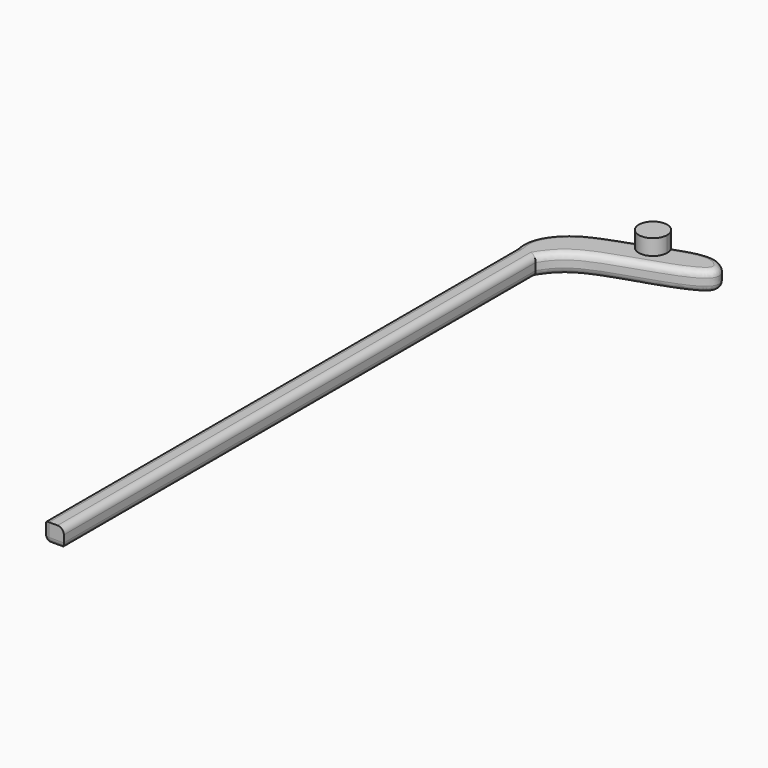
from build123d import *

# Parameters (mm, degrees)
F0_W     = 6.8017598242
F0_H     = 190.8443272114
F1_DEPTH = 6.35
F2_R     = 2.032
F4_DEPTH = 5.08


with BuildPart() as f1:
    # F0 (on Top) → F1 (new body)
    with BuildSketch(Plane.XY):
        with BuildLine():
            add(Edge.make_bspline(
                [(-18.7212117016, 95.2281802893), (-19.0287577276, 97.276144289), (-19.7432919814, 102.0342608203), (-12.2874624611, 112.4930440931), (5.2710494303, 117.2298121441), (24.2765167775, 126.2039152993), (34.1874650886, 113.5896617546), (-5.0813319368, 105.699253631), (-10.0400502329, 98.10603191), (-11.9194518775, 95.2281802893)],
                knots=[0, 0, 0, 0, 0.0947219775, 0.2200713026, 0.3846456115, 0.5513063344, 0.6487683321, 0.8668823782, 1, 1, 1, 1], degree=3))
            Line((-18.7212117016, 95.2281802893), (-11.9194518775, 95.2281802893))
        make_face()
        with Locations((-15.3203317896, -0.1939833164)):
            Rectangle(F0_W, F0_H)
    extrude(amount=F1_DEPTH)

    # F2
    f2_edges = [f1.edges().sort_by_distance(p)[0] for p in [
        (-11.919452, -0.193983, 0),
        (23.633961, 122.958027, 0),
        (-15.320332, -95.616147, 0),
        (-18.721212, -0.193983, 0),
        (-18.721212, 95.22818, 3.175),
        (-18.721212, -95.616147, 3.175),
        (-18.721212, -0.193983, 6.35),
        (-11.919452, -0.193983, 6.35),
        (19.705715, 122.814147, 6.35),
    ]]
    fillet(f2_edges, radius=F2_R)

    # F3 (on face) → F4 (join)
    with BuildSketch(Plane.XY.offset(6.35)):
        with BuildLine():
            add(Edge.make_bspline(
                [(4.3073198253, 115.4028172782), (4.4655770028, 115.4600073559), (4.6241664565, 115.5174753315), (4.7830828302, 115.5752301503), (4.9423207723, 115.633280776), (5.1018749356, 115.6916361901), (5.2617399779, 115.7503053906), (5.4219105623, 115.809297391), (5.5823813583, 115.8686212189), (5.7431470418, 115.9282859145), (5.9042022968, 115.9883005294), (6.065541816, 116.0486741248), (6.2271603024, 116.1094157692), (6.891473352, 116.3602123058), (7.3942257017, 116.5526503246), (7.897031711, 116.7472316138), (8.3996299922, 116.943343569), (8.9017468193, 117.1403738641), (9.4030911518, 117.3377101569), (9.9033572408, 117.5347404905), (10.4022278152, 117.730853482), (10.899375726, 117.9254383095), (11.3944640632, 118.1178847226), (11.8871453472, 118.3075832528), (12.3770603156, 118.4939257109), (12.8638365931, 118.676306045)],
                knots=[41.1069525141, 41.1069525141, 41.1069525141, 41.1069525141, 41.1069525141, 41.1069525141, 41.1069525141, 41.1069525141, 41.1069525141, 41.1069525141, 41.1069525141, 41.1069525141, 41.1069525141, 41.1069525141, 42.9706736291, 42.9706736291, 42.9706736291, 42.9706736291, 42.9706736291, 42.9706736291, 42.9706736291, 42.9706736291, 42.9706736291, 42.9706736291, 42.9706736291, 42.9706736291, 48.7546001647, 48.7546001647, 48.7546001647, 48.7546001647, 48.7546001647, 48.7546001647, 48.7546001647, 48.7546001647, 48.7546001647, 48.7546001647, 48.7546001647, 48.7546001647, 48.7546001647, 48.7546001647], degree=13))
            ThreePointArc((12.8638365931, 118.676306045), (6.956170165, 121.2986437127), (4.3073198253, 115.4028172782))
        make_face()
        with BuildLine():
            ThreePointArc((4.3073198253, 115.4028172782), (9.4150421515, 112.5140150742), (13.1736352055, 117.0203421585))
            ThreePointArc((13.1736352055, 117.0203421585), (13.0955194905, 117.8626888172), (12.8638365931, 118.676306045))
            add(Edge.make_bspline(
                [(4.3073198253, 115.4028172782), (4.4655770028, 115.4600073559), (4.6241664565, 115.5174753315), (4.7830828302, 115.5752301503), (4.9423207723, 115.633280776), (5.1018749356, 115.6916361901), (5.2617399779, 115.7503053906), (5.4219105623, 115.809297391), (5.5823813583, 115.8686212189), (5.7431470418, 115.9282859145), (5.9042022968, 115.9883005294), (6.065541816, 116.0486741248), (6.2271603024, 116.1094157692), (6.891473352, 116.3602123058), (7.3942257017, 116.5526503246), (7.897031711, 116.7472316138), (8.3996299922, 116.943343569), (8.9017468193, 117.1403738641), (9.4030911518, 117.3377101569), (9.9033572408, 117.5347404905), (10.4022278152, 117.730853482), (10.899375726, 117.9254383095), (11.3944640632, 118.1178847226), (11.8871453472, 118.3075832528), (12.3770603156, 118.4939257109), (12.8638365931, 118.676306045)],
                knots=[41.1069525141, 41.1069525141, 41.1069525141, 41.1069525141, 41.1069525141, 41.1069525141, 41.1069525141, 41.1069525141, 41.1069525141, 41.1069525141, 41.1069525141, 41.1069525141, 41.1069525141, 41.1069525141, 42.9706736291, 42.9706736291, 42.9706736291, 42.9706736291, 42.9706736291, 42.9706736291, 42.9706736291, 42.9706736291, 42.9706736291, 42.9706736291, 42.9706736291, 42.9706736291, 48.7546001647, 48.7546001647, 48.7546001647, 48.7546001647, 48.7546001647, 48.7546001647, 48.7546001647, 48.7546001647, 48.7546001647, 48.7546001647, 48.7546001647, 48.7546001647, 48.7546001647, 48.7546001647], degree=13))
        make_face()
    extrude(amount=F4_DEPTH)


solid = f1.part
